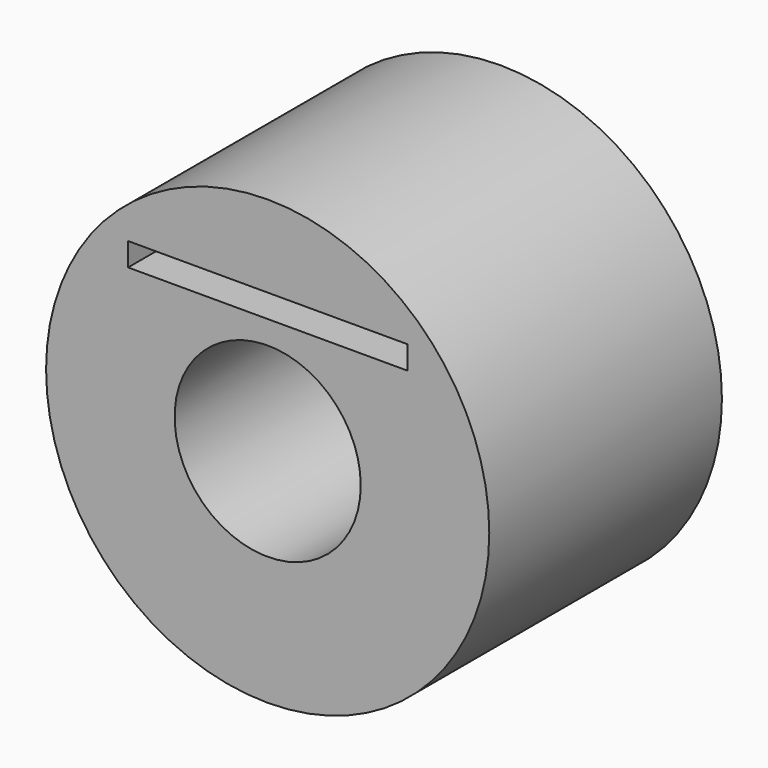
from build123d import *

# Parameters (mm, degrees)
F0_R     = 19.05
F0_R_2   = 8
F0_W     = 24
F0_H     = 2
F3_DEPTH = 25


# Not quite as in the source:
# - the program builds the solid bodies; features that only make, move or delete a surface that nothing else refers to are left out


with BuildPart() as f3:
    # F0 (on Front) → F3 (new body)
    with BuildSketch(Plane.XZ):
        Circle(F0_R)
        Circle(F0_R_2, mode=Mode.SUBTRACT)
        with Locations((0, 11)):
            Rectangle(F0_W, F0_H, mode=Mode.SUBTRACT)
    extrude(amount=F3_DEPTH)


solid = f3.part
